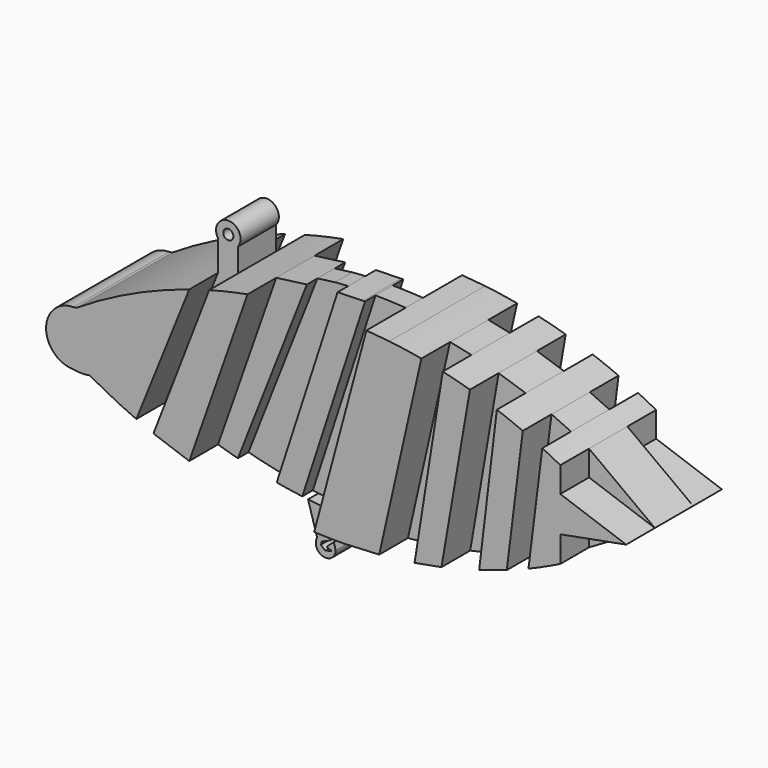
from build123d import *

# Parameters (mm, degrees)
F1_DEPTH = 6.35
F2_DEPTH = 1.143
F0_R     = 0.5376774343
F3_DEPTH = 2.54


# Not quite as in the source:
# - a feature names something its author has since deleted; it is built from what else it names


with BuildPart() as f1:
    # F0 (on Front) → F1 (new body, symmetric)
    with BuildSketch(Plane.XZ):
        with BuildLine():
            Line((-23.957899441, 10.4580381471), (-18.3417778462, 24.3978608632))
            ThreePointArc((-18.3417778462, 24.3978608632), (-24.508682548, 21.9832418882), (-30.3090570475, 18.7868761299))
            ThreePointArc((-30.3090570475, 18.7868761299), (-30.4688345425, 18.7669734191), (-30.6283324456, 18.7449419699))
            ThreePointArc((-30.6283324456, 18.7449419699), (-33.5331514259, 15.8401229896), (-30.6283324456, 12.9353040093))
            ThreePointArc((-30.6283324456, 12.9353040093), (-29.7623700905, 12.8471763438), (-28.8964077355, 12.9353040093))
            ThreePointArc((-28.8964077355, 12.9353040093), (-26.4593844973, 11.6324177359), (-23.957899441, 10.4580381471))
        make_face()
    extrude(amount=F1_DEPTH, both=True)



with BuildPart() as f1b:
    # F0 (on Front) → F1, piece 2 (new body, symmetric)
    with BuildSketch(Plane.XZ):
        with BuildLine():
            Line((-18.3417778462, 8.3667041198), (-12.1646409942, 25.9439263056))
            ThreePointArc((-12.1646409942, 25.9439263056), (-14.2076271577, 25.5232665303), (-16.2316225469, 25.0190941641))
            Line((-16.2316225469, 25.0190941641), (-22.1410569955, 9.7018790977))
            Line((-22.1410569955, 9.7018790977), (-18.3417778462, 8.3667041198))
        make_face()
    extrude(amount=F1_DEPTH, both=True)


with BuildPart() as f1c:
    # F0 (on Front) → F1, piece 3 (new body, symmetric)
    with BuildSketch(Plane.XZ):
        with BuildLine():
            Line((1.8068482134, 6.1805279437), (6.278092768, 25.9439263056))
            ThreePointArc((6.278092768, 25.9439263056), (4.5833562732, 26.2272072808), (2.8800089407, 26.4530119809))
            Line((2.8800089407, 26.4530119809), (-1.8782013648, 5.999318733))
            Line((-1.8782013648, 5.999318733), (1.8068482134, 6.1805279437))
        make_face()
        with BuildLine():
            Line((-1.8782013648, 5.999318733), (2.8800089407, 26.4530119809))
            Line((2.8800089407, 26.4530119809), (0.4476490102, 26.6745825214))
            Line((0.4476490102, 26.6745825214), (-5.0909425313, 6.0502526163))
            ThreePointArc((-5.0909425313, 6.0502526163), (-3.4849571687, 6.0004872294), (-1.8782013648, 5.999318733))
        make_face()
    extrude(amount=F1_DEPTH, both=True)


with BuildPart() as f1d:
    # F0 (on Front) → F1, piece 4 (new body, symmetric)
    with BuildSketch(Plane.XZ):
        with BuildLine():
            Line((8.4127366642, 7.1570997269), (11.4288211982, 24.7124430234))
            ThreePointArc((11.4288211982, 24.7124430234), (9.992896211, 25.1131857412), (8.5458304529, 25.4716212117))
            Line((8.5458304529, 25.4716212117), (5.5570962218, 6.6305751818))
            Line((5.5570962218, 6.6305751818), (8.4127366642, 7.1570997269))
        make_face()
    extrude(amount=F1_DEPTH, both=True)


with BuildPart() as f1e:
    # F0 (on Front) → F1, piece 5 (new body, symmetric)
    with BuildSketch(Plane.XZ):
        with BuildLine():
            Line((15.3388230563, 9.1300772804), (17.0374851182, 22.6934409017))
            ThreePointArc((17.0374851182, 22.6934409017), (15.6698818595, 23.2551052755), (14.2865132328, 23.7767342476))
            Line((14.2865132328, 23.7767342476), (12.4090739429, 8.1711044117))
            Line((12.4090739429, 8.1711044117), (15.3388230563, 9.1300772804))
        make_face()
    extrude(amount=F1_DEPTH, both=True)


with BuildPart() as f1f:
    # F0 (on Front) → F1, piece 6 (new body, symmetric)
    with BuildSketch(Plane.XZ):
        with BuildLine():
            Line((21.0198694331, 18.0883333087), (21.0198694322, 20.7808247964))
            ThreePointArc((21.0198694322, 20.7808247964), (20.069859076, 21.2762433466), (19.1096116707, 21.7515160445))
            Line((19.1096116707, 21.7515160445), (17.6402366731, 10.0189484933))
            ThreePointArc((17.6402366731, 10.0189484933), (19.3434832269, 10.757776133), (21.0198694351, 11.5556761172))
            Line((21.0198694351, 11.5556761172), (21.0198694343, 14.3284648657))
            Line((21.0198694343, 14.3284648657), (21.0198694331, 18.0883333087))
        make_face()
        Polygon((21.0198694343, 14.3284648657), (28.0039037731, 15.6337103452), (21.0198694331, 18.0883333087), align=None)
    extrude(amount=F1_DEPTH, both=True)


with BuildPart() as f1_1:
    add(f1.part)

    add(f1b.part)  # F2 merges F1b

    add(f1c.part)  # F2 merges F1c

    add(f1d.part)  # F2 merges F1d

    add(f1e.part)  # F2 merges F1e

    add(f1f.part)  # F2 merges F1f
    # F0 (on Front) → F2 (join, symmetric)
    with BuildSketch(Plane.XZ):
        with BuildLine():
            Line((-12.1127719974, 6.8447730539), (-5.6567463208, 26.7153601349))
            ThreePointArc((-5.6567463208, 26.7153601349), (-6.3478066879, 26.6736702184), (-7.0382347309, 26.6225664263))
            Line((-7.0382347309, 26.6225664263), (-8.9119801903, 26.3745176413))
            Line((-8.9119801903, 26.3745176413), (-16.2316225469, 7.7613705689))
            ThreePointArc((-16.2316225469, 7.7613705689), (-14.1813025903, 7.2621558762), (-12.1127719974, 6.8447730539))
        make_face()
        with BuildLine():
            Line((-5.0909425313, 6.0502526163), (0.4476490102, 26.6745825214))
            ThreePointArc((0.4476490102, 26.6745825214), (-1.1501754418, 26.7562261377), (-2.7497784488, 26.787513187))
            Line((-2.7497784488, 26.787513187), (-9.4000246121, 6.4253498282))
            ThreePointArc((-9.4000246121, 6.4253498282), (-9.0947770245, 6.3870993561), (-8.7893130258, 6.3506173901))
            ThreePointArc((-8.7893130258, 6.3506173901), (-7.91449717, 6.2560428931), (-7.0382347309, 6.1759725811))
            ThreePointArc((-7.0382347309, 6.1759725811), (-6.0651659933, 6.1041697642), (-5.0909425313, 6.0502526163))
        make_face()
        with BuildLine():
            Line((-9.4000246121, 6.4253498282), (-2.7497784488, 26.787513187))
            ThreePointArc((-2.7497784488, 26.787513187), (-2.8593531847, 26.7878123797), (-2.968928311, 26.7878752202))
            Line((-2.968928311, 26.7878752202), (-5.6567463208, 26.7153601349))
            Line((-5.6567463208, 26.7153601349), (-12.1127719974, 6.8447730539))
            ThreePointArc((-12.1127719974, 6.8447730539), (-10.7591081046, 6.6175349855), (-9.4000246121, 6.4253498282))
        make_face()
        with BuildLine():
            ThreePointArc((-18.3417778462, 8.3667041198), (-17.2898277228, 8.0531349816), (-16.2316225469, 7.7613705689))
            Line((-16.2316225469, 7.7613705689), (-8.9119801903, 26.3745176413))
            Line((-8.9119801903, 26.3745176413), (-12.1646409942, 25.9439263056))
            Line((-12.1646409942, 25.9439263056), (-18.3417778462, 8.3667041198))
        make_face()
        with BuildLine():
            Line((5.5570962218, 6.6305751818), (8.5458304529, 25.4716212117))
            Line((8.5458304529, 25.4716212117), (6.278092768, 25.9439263056))
            Line((6.278092768, 25.9439263056), (1.8068482134, 6.1805279437))
            ThreePointArc((1.8068482134, 6.1805279437), (3.6859738146, 6.3722062161), (5.5570962218, 6.6305751818))
        make_face()
        with BuildLine():
            Line((12.4090739429, 8.1711044117), (14.2865132328, 23.7767342476))
            Line((14.2865132328, 23.7767342476), (11.4288211982, 24.7124430234))
            Line((11.4288211982, 24.7124430234), (8.4127366642, 7.1570997269))
            ThreePointArc((8.4127366642, 7.1570997269), (10.4207473928, 7.62531299), (12.4090739429, 8.1711044117))
        make_face()
        with BuildLine():
            Line((17.6402366731, 10.0189484933), (19.1096116707, 21.7515160445))
            Line((19.1096116707, 21.7515160445), (17.0374851182, 22.6934409017))
            Line((17.0374851182, 22.6934409017), (15.3388230563, 9.1300772804))
            ThreePointArc((15.3388230563, 9.1300772804), (16.4946911486, 9.5611495909), (17.6402366731, 10.0189484933))
        make_face()
        with BuildLine():
            Line((-22.1410569955, 9.7018790977), (-16.2316225469, 25.0190941641))
            ThreePointArc((-16.2316225469, 25.0190941641), (-17.2900631098, 24.7199003867), (-18.3417778462, 24.3978608632))
            Line((-18.3417778462, 24.3978608632), (-23.957899441, 10.4580381471))
            ThreePointArc((-23.957899441, 10.4580381471), (-23.0529803303, 10.0715440095), (-22.1410569955, 9.7018790977))
        make_face()
    extrude(amount=F2_DEPTH, both=True)

    # F0 (on Front) → F3 (join, symmetric)
    with BuildSketch(Plane.XZ):
        with BuildLine():
            Line((-22.1410569955, 9.7018790977), (-16.2316225469, 25.0190941641))
            ThreePointArc((-16.2316225469, 25.0190941641), (-17.2900631098, 24.7199003867), (-18.3417778462, 24.3978608632))
            Line((-18.3417778462, 24.3978608632), (-23.957899441, 10.4580381471))
            ThreePointArc((-23.957899441, 10.4580381471), (-23.0529803303, 10.0715440095), (-22.1410569955, 9.7018790977))
        make_face()
        with BuildLine():
            ThreePointArc((-18.3417778462, 8.3667041198), (-17.2898277228, 8.0531349816), (-16.2316225469, 7.7613705689))
            Line((-16.2316225469, 7.7613705689), (-8.9119801903, 26.3745176413))
            Line((-8.9119801903, 26.3745176413), (-12.1646409942, 25.9439263056))
            Line((-12.1646409942, 25.9439263056), (-18.3417778462, 8.3667041198))
        make_face()
        with BuildLine():
            Line((-9.4000246121, 6.4253498282), (-2.7497784488, 26.787513187))
            ThreePointArc((-2.7497784488, 26.787513187), (-2.8593531847, 26.7878123797), (-2.968928311, 26.7878752202))
            Line((-2.968928311, 26.7878752202), (-5.6567463208, 26.7153601349))
            Line((-5.6567463208, 26.7153601349), (-12.1127719974, 6.8447730539))
            ThreePointArc((-12.1127719974, 6.8447730539), (-10.7591081046, 6.6175349855), (-9.4000246121, 6.4253498282))
        make_face()
        with BuildLine():
            Line((5.5570962218, 6.6305751818), (8.5458304529, 25.4716212117))
            Line((8.5458304529, 25.4716212117), (6.278092768, 25.9439263056))
            Line((6.278092768, 25.9439263056), (1.8068482134, 6.1805279437))
            ThreePointArc((1.8068482134, 6.1805279437), (3.6859738146, 6.3722062161), (5.5570962218, 6.6305751818))
        make_face()
        with BuildLine():
            Line((12.4090739429, 8.1711044117), (14.2865132328, 23.7767342476))
            Line((14.2865132328, 23.7767342476), (11.4288211982, 24.7124430234))
            Line((11.4288211982, 24.7124430234), (8.4127366642, 7.1570997269))
            ThreePointArc((8.4127366642, 7.1570997269), (10.4207473928, 7.62531299), (12.4090739429, 8.1711044117))
        make_face()
        with BuildLine():
            Line((17.6402366731, 10.0189484933), (19.1096116707, 21.7515160445))
            Line((19.1096116707, 21.7515160445), (17.0374851182, 22.6934409017))
            Line((17.0374851182, 22.6934409017), (15.3388230563, 9.1300772804))
            ThreePointArc((15.3388230563, 9.1300772804), (16.4946911486, 9.5611495909), (17.6402366731, 10.0189484933))
        make_face()
        Polygon((28.0039037731, 15.6337103452), (21.0198694322, 20.7808247964), (21.0198694331, 18.0883333087), align=None)
        Polygon((21.0198694351, 11.5556761172), (28.0039037731, 15.6337103452), (21.0198694343, 14.3284648657), align=None)
        with BuildLine():
            ThreePointArc((-18.3417778462, 24.3978608632), (-17.2900631098, 24.7199003867), (-16.2316225469, 25.0190941641))
            Line((-16.2316225469, 25.0190941641), (-16.2316225469, 27.5203254709))
            Line((-16.2316225469, 27.5203254709), (-18.3417778462, 27.6264417917))
            Line((-18.3417778462, 27.6264417917), (-18.3417778462, 24.3978608632))
        make_face()
        with BuildLine():
            Line((-18.3417778462, 27.6264417917), (-16.2316225469, 27.5203254709))
            ThreePointArc((-16.2316225469, 27.5203254709), (-17.1834027814, 29.6274841361), (-18.3417778462, 27.6264417917))
        make_face()
        with Locations((-17.248678008, 28.3294664105)):
            Circle(F0_R, mode=Mode.SUBTRACT)
        with BuildLine():
            Line((-6.263176576, 3.5358044787), (-7.0382347309, 6.1759725811))
            ThreePointArc((-7.0382347309, 6.1759725811), (-7.91449717, 6.2560428931), (-8.7893130258, 6.3506173901))
            Line((-8.7893130258, 6.3506173901), (-7.8281190425, 3.0763937997))
            Line((-7.8281190425, 3.0763937997), (-6.263176576, 3.5358044787))
        make_face()
        with BuildLine():
            Line((-6.4755459316, 3.2506433781), (-6.263176576, 3.5358044787))
            Line((-6.263176576, 3.5358044787), (-7.8281190425, 3.0763937997))
            ThreePointArc((-7.8281190425, 3.0763937997), (-7.1834055221, 1.5302282542), (-5.857669426, 2.5542923249))
            Line((-5.857669426, 2.5542923249), (-6.0594304827, 3.2415737925))
            Line((-6.0594304827, 3.2415737925), (-6.6755125299, 2.7018676046))
            Line((-6.6755125299, 2.7018676046), (-6.8233669735, 2.54364172))
            Line((-6.8233669735, 2.54364172), (-6.2799803729, 2.3477658746))
            Line((-6.2799803729, 2.3477658746), (-6.9631087507, 2.1509963489))
            Line((-6.9631087507, 2.1509963489), (-7.4357455596, 2.5542923249))
            Line((-7.4357455596, 2.5542923249), (-7.3302290402, 2.8919170145))
            Line((-7.3302290402, 2.8919170145), (-6.4755459316, 3.2506433781))
        make_face()
    extrude(amount=F3_DEPTH, both=True)


solid = f1_1.part
